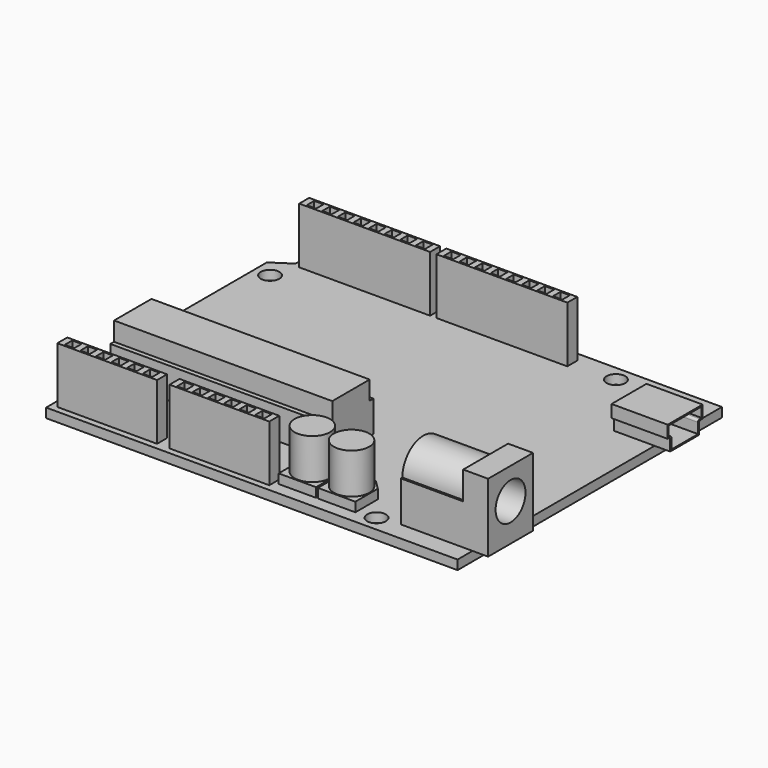
from build123d import *

# Parameters (mm, degrees)
F0_R          = 1.5
F0_W          = 11.5
F0_H          = 9
F1_DEPTH      = 1.5
F2_W          = 21
F2_H          = 2
F2_W_2        = 16
F3_DEPTH      = 9
F4_W          = 1.5
F4_H          = 1.5
F5_DEPTH      = 6
F6_W          = 1.5
F6_H          = 1.5
F7_DEPTH      = 6
F8_W          = 1.5
F8_H          = 1.5
F9_DEPTH      = 6
F10_W         = 1.5
F10_H         = 1.5
F11_DEPTH     = 6
F13_DEPTH     = 1.5
F15_R         = 2.85
F14_R         = 2.85
F16_DEPTH     = 6.5
F17_W         = 14
F17_H         = 9
F18_DEPTH     = 11
F20_DEPTH     = 10
F21_R         = 3
F22_DEPTH     = 12.5
F23_W         = 6.5
F23_H         = 7
F23_W_2       = 2.5
F24_DEPTH     = 4
F26_DEPTH     = 10
F28_DEPTH     = 7.5
F29_W         = 35
F29_H         = 9
F30_DEPTH     = 5
F31_W         = 35
F31_H         = 7.5
F32_DEPTH     = 3
F33_TEXT_SIZE = 6.9665593199
F34_DEPTH     = 0.5


# Not quite as in the source:
# - Text() gives the source's letters only with a copy of the font that has no kerning and outlines rounded to 1/6400 em; it was checked with that copy


with BuildPart() as f1:
    # F0 (on Top) → F1 (new body)
    with BuildSketch(Plane.XY):
        Polygon((24.8085663617, 53), (-41.1914336383, 53), (-41.1914336383, 50), (-44.1914336383, 48.0100251258), (-44.1914336383, 15.0100251258), (-41.1914336383, 13), (-41.1914336383, 12.5659361547), (-41.1914336383, 0), (24.8085663617, 0), (24.8085663617, 3), (13.3085663617, 3), (13.3085663617, 12), (24.8085663617, 12), align=None)
        with BuildLine():
            ThreePointArc((-41.6914336383, 18.972135955), (-40.6307734666, 18.5327961268), (-40.1914336383, 17.472135955))
            ThreePointArc((-40.1914336383, 17.472135955), (-42.7520938101, 16.4114757832), (-41.6914336383, 18.972135955))
        make_face(mode=Mode.SUBTRACT)
        with Locations((9.8085663617, 2.5)):
            Circle(F0_R, mode=Mode.SUBTRACT)
        with Locations((-41.6914336383, 45.527864045)):
            Circle(F0_R, mode=Mode.SUBTRACT)
        with Locations((9.8085663617, 50.5)):
            Circle(F0_R, mode=Mode.SUBTRACT)
        with Locations((19.0585663617, 7.5)):
            Rectangle(F0_W, F0_H)
    extrude(amount=F1_DEPTH)

    # F2 (on face) → F3 (join)
    with BuildSketch(Plane.XY.offset(1.5)):
        with Locations((-7.6914336383, 50.5)):
            Rectangle(F2_W, F2_H)
        with Locations((-29.6914336383, 50.5)):
            Rectangle(F2_W, F2_H)
        with Locations((-14.1914336383, 2)):
            Rectangle(F2_W_2, F2_H)
        with Locations((-32.1914336383, 2)):
            Rectangle(F2_W_2, F2_H)
    extrude(amount=F3_DEPTH)

    # F4 (on face) → F5 (cut)
    with BuildSketch(Plane.XY.offset(10.5)):
        with Locations((-38.4414336383, 50.5)):
            Rectangle(F4_W, F4_H)
        with Locations((-35.9414336383, 50.5)):
            Rectangle(F4_W, F4_H)
        with Locations((-33.4414336383, 50.5)):
            Rectangle(F4_W, F4_H)
        with Locations((-30.9414336383, 50.5)):
            Rectangle(F4_W, F4_H)
        with Locations((-28.4414336383, 50.5)):
            Rectangle(F4_W, F4_H)
        with Locations((-25.9414336383, 50.5)):
            Rectangle(F4_W, F4_H)
        with Locations((-20.9414336383, 50.5)):
            Rectangle(F4_W, F4_H)
        with Locations((-23.4414336383, 50.5)):
            Rectangle(F4_W, F4_H)
    extrude(amount=-F5_DEPTH, mode=Mode.SUBTRACT)

    # F6 (on face) → F7 (cut)
    with BuildSketch(Plane.XY.offset(10.5)):
        with Locations((-13.9414336383, 50.5)):
            Rectangle(F6_W, F6_H)
        with Locations((-11.4414336383, 50.5)):
            Rectangle(F6_W, F6_H)
        with Locations((-8.9414336383, 50.5)):
            Rectangle(F6_W, F6_H)
        with Locations((-6.4414336383, 50.5)):
            Rectangle(F6_W, F6_H)
        with Locations((-3.9414336383, 50.5)):
            Rectangle(F6_W, F6_H)
        with Locations((1.0585663617, 50.5)):
            Rectangle(F6_W, F6_H)
        with Locations((-1.4414336383, 50.5)):
            Rectangle(F6_W, F6_H)
        with Locations((-16.4414336383, 50.5)):
            Rectangle(F6_W, F6_H)
    extrude(amount=-F7_DEPTH, mode=Mode.SUBTRACT)

    # F8 (on face) → F9 (cut)
    with BuildSketch(Plane.XY.offset(10.5)):
        with Locations((-38.4414336383, 2)):
            Rectangle(F8_W, F8_H)
        with Locations((-35.9414336383, 2)):
            Rectangle(F8_W, F8_H)
        with Locations((-33.4414336383, 2)):
            Rectangle(F8_W, F8_H)
        with Locations((-30.9414336383, 2)):
            Rectangle(F8_W, F8_H)
        with Locations((-28.4414336383, 2)):
            Rectangle(F8_W, F8_H)
        with Locations((-25.9414336383, 2)):
            Rectangle(F8_W, F8_H)
    extrude(amount=-F9_DEPTH, mode=Mode.SUBTRACT)

    # F10 (on face) → F11 (cut)
    with BuildSketch(Plane.XY.offset(10.5)):
        with Locations((-20.4414336383, 2)):
            Rectangle(F10_W, F10_H)
        with Locations((-17.9414336383, 2)):
            Rectangle(F10_W, F10_H)
        with Locations((-15.4414336383, 2)):
            Rectangle(F10_W, F10_H)
        with Locations((-12.9414336383, 2)):
            Rectangle(F10_W, F10_H)
        with Locations((-10.4414336383, 2)):
            Rectangle(F10_W, F10_H)
        with Locations((-7.9414336383, 2)):
            Rectangle(F10_W, F10_H)
    extrude(amount=-F11_DEPTH, mode=Mode.SUBTRACT)

    # F12 (on face) → F13 (join)
    with BuildSketch(Plane.XY.offset(1.5)):
        Polygon((5.3085663617, 8), (2.3085663617, 8), (0.8085663617, 6.5), (0.8085663617, 2), (6.8085663617, 2), (6.8085663617, 6.5), align=None)
        Polygon((0.5085663617, 6.5), (-0.9914336383, 8), (-3.9914336383, 8), (-5.4914336383, 6.5), (-5.4914336383, 2), (0.5085663617, 2), align=None)
    extrude(amount=F13_DEPTH)

    # F15 (on face) + F14 (on face) → F16 (join)
    with BuildSketch(Plane.XY.offset(3)):
        with Locations((3.8085663617, 5)):
            Circle(F15_R)
    with BuildSketch(Plane.XY.offset(3)):
        with Locations((-2.4914336383, 5)):
            Circle(F14_R)
    extrude(amount=F16_DEPTH)

    # F17 (on face) → F18 (join)
    with BuildSketch(Plane.XY.offset(1.5)):
        with Locations((20.3085663617, 7.5)):
            Rectangle(F17_W, F17_H)
    extrude(amount=F18_DEPTH)

    # F19 (on face) → F20 (cut)
    with BuildSketch(Plane(origin=(13.3085663617, 0, 0), x_dir=(0, -1, 0), z_dir=(-1, 0, 0))):
        with BuildLine():
            Line((-12, 8), (-11.7, 8))
            ThreePointArc((-11.7, 8), (-7.5, 12.2), (-3.3, 8))
            Line((-3.3, 8), (-3, 8))
            Line((-3, 8), (-3, 12.5))
            Line((-3, 12.5), (-12, 12.5))
            Line((-12, 12.5), (-12, 8))
        make_face()
    extrude(amount=-F20_DEPTH, mode=Mode.SUBTRACT)

    # F21 (on face) → F22 (cut)
    with BuildSketch(Plane.YZ.offset(27.3085663617)):
        with Locations((7.5, 7.5)):
            Circle(F21_R)
    extrude(amount=-F22_DEPTH, mode=Mode.SUBTRACT)

    # F23 (on face) → F24 (join)
    with BuildSketch(Plane.XY.offset(1.5)):
        with Locations((21.5585663617, 42.5)):
            Rectangle(F23_W, F23_H)
        with Locations((26.0585663617, 42.5)):
            Rectangle(F23_W_2, F23_H)
    extrude(amount=F24_DEPTH)

    # F25 (on face) → F26 (cut)
    with BuildSketch(Plane.YZ.offset(27.3085663617)):
        with BuildLine():
            Line((39.35, 3.5), (39, 3.5))
            Line((39, 3.5), (39, 1.5))
            Line((39, 1.5), (39.5, 1.5))
            Line((39.5, 1.5), (39.5, 3.35))
            ThreePointArc((39.5, 3.35), (39.4289887257, 3.4289887257), (39.35, 3.5))
        make_face()
        with BuildLine():
            Line((46, 1.5), (46, 3.5))
            Line((46, 3.5), (45.434692198, 3.5))
            ThreePointArc((45.434692198, 3.5), (45.3557034724, 3.4289887257), (45.284692198, 3.35))
            Line((45.284692198, 3.35), (45.284692198, 1.5))
            Line((45.284692198, 1.5), (46, 1.5))
        make_face()
    extrude(amount=-F26_DEPTH, mode=Mode.SUBTRACT)

    # F27 (on face) → F28 (cut)
    with BuildSketch(Plane.YZ.offset(27.3085663617)):
        with BuildLine():
            Line((45.8, 5.3), (39.2, 5.3))
            Line((39.2, 5.3), (39.2, 3.7))
            Line((39.2, 3.7), (39.35, 3.7))
            ThreePointArc((39.35, 3.7), (39.6157536453, 3.6001470232), (39.75, 3.35))
            Line((39.75, 3.35), (39.75, 1.7))
            Line((39.75, 1.7), (45.084692198, 1.7))
            Line((45.084692198, 1.7), (45.084692198, 3.35))
            ThreePointArc((45.084692198, 3.35), (45.1893513969, 3.5953408011), (45.434692198, 3.7))
            Line((45.434692198, 3.7), (45.8, 3.7))
            Line((45.8, 3.7), (45.8, 5.3))
        make_face()
    extrude(amount=-F28_DEPTH, mode=Mode.SUBTRACT)

    # F29 (on face) → F30 (join)
    with BuildSketch(Plane.XY.offset(1.5)):
        with Locations((-22.1914336383, 15.5)):
            Rectangle(F29_W, F29_H)
    extrude(amount=F30_DEPTH)

    # F31 (on face) → F32 (join)
    with BuildSketch(Plane.XY.offset(6.5)):
        with Locations((-22.1914336383, 15.5)):
            Rectangle(F31_W, F31_H)
    extrude(amount=F32_DEPTH)

    # F33 (on face) → F34 (join)
    with BuildSketch(Plane(origin=(0, 0, 0), x_dir=(1, 0, 0), z_dir=(0, 0, -1))):
        with Locations((-32.4363075197, -14.2117831856)):
            Text('Annie Zhu', F33_TEXT_SIZE, font='Open Sans', text_align=(TextAlign.LEFT, TextAlign.BOTTOM))
        with Locations((-32.4363075197, -23.6863038606)):
            Text('Kathy Kang', F33_TEXT_SIZE, font='Open Sans', text_align=(TextAlign.LEFT, TextAlign.BOTTOM))
    extrude(amount=F34_DEPTH)


solid = f1.part
